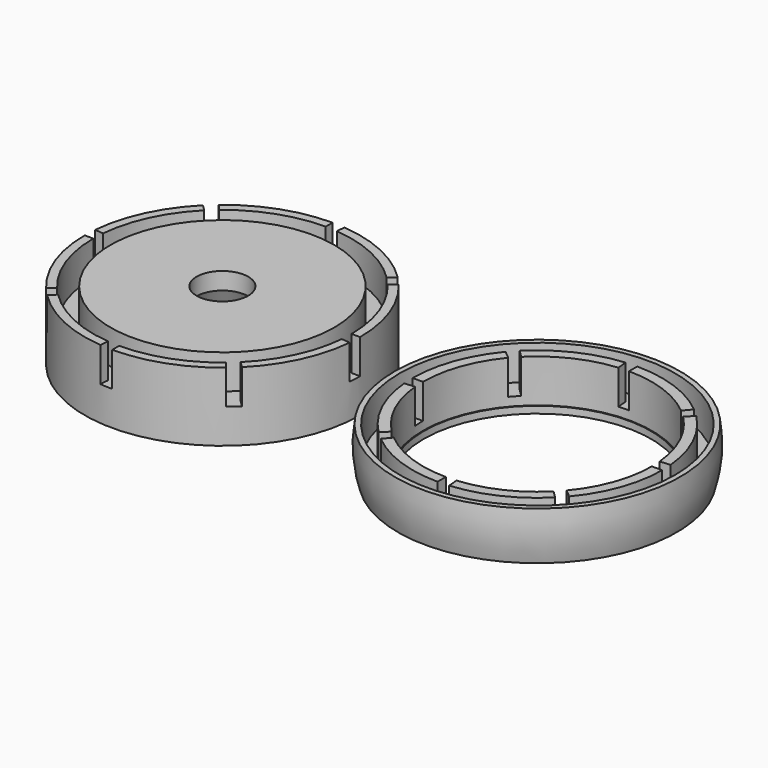
from build123d import *

# Parameters (mm, degrees)
F3_DEPTH        = 2.54
F3_COPIES_COUNT = 8
F7_DEPTH        = 2.54
F7_COPIES_COUNT = 8


# Not quite as in the source:
# - a pattern or mirror of a feature is missing from the dataset's text; its kind, count and spacing are read off the source's solid


with BuildPart() as f1:
    # F0 (on Front) → F1 (revolve)
    with BuildSketch(Plane.XZ):
        Polygon((-6.35, 0), (0, 0), (0, 5.08), (-0.635, 5.08), (-0.635, 2.54), (-1.905, 2.54), (-1.905, 5.08), (-8.255, 5.08), (-8.255, 3.81), align=None)
    revolve(axis=Axis((-10.16, 0, 2.5961052161), (0, 0, 1)))

    # F2 (on face) → F3 (cut, through all)
    with BuildSketch(Plane.XY.offset(5.08)):
        with BuildLine():
            ThreePointArc((-0.635, 0), (-0.6445944791, -0.4274140533), (-0.6733585875, -0.853967043))
            Line((-0.6733585875, -0.853967043), (-0.0409158267, -0.9108981792))
            ThreePointArc((-0.0409158267, -0.9108981792), (-0.010234111, -0.4559083235), (0, 0))
            Line((0, 0), (-0.635, 0))
        make_face()
    f3 = extrude(amount=-F3_DEPTH, mode=Mode.SUBTRACT)

    # F3_copies: F3 ×8 about axis
    f3_copies_axis = Axis((-10.16, 0, 0), (0, 0, 1))
    for i in range(1, F3_COPIES_COUNT):
        add(f3.rotate(f3_copies_axis, i * 360 / F3_COPIES_COUNT), mode=Mode.SUBTRACT)


with BuildPart() as f5:
    # F4 (on Front) → F5 (revolve)
    with BuildSketch(Plane.XZ):
        with BuildLine():
            Line((2.794, 0), (4.699, 0))
            Line((4.699, 0), (4.699, 0.508))
            Line((4.699, 0.508), (4.6355, 0.508))
            Line((4.6355, 0.508), (4.6355, 3.683))
            Line((4.6355, 3.683), (3.8735, 3.683))
            Line((3.8735, 3.683), (3.8735, 1.143))
            Line((3.8735, 1.143), (2.921, 1.143))
            Line((2.921, 1.143), (2.921, 3.683))
            Line((2.921, 3.683), (2.54, 3.683))
            ThreePointArc((2.54, 3.683), (2.4478454241, 1.8263858913), (2.794, 0))
        make_face()
    revolve(axis=Axis((13.081, 0, 1.3761192095), (0, 0, 1)))

    # F6 (on face) → F7 (cut, through all)
    with BuildSketch(Plane.XY.offset(3.683)):
        with BuildLine():
            ThreePointArc((12.3236263902, 8.4114716587), (12.7019311696, 8.4369886258), (13.081, 8.4455))
            Line((13.081, 8.4455), (13.081, 9.2075))
            ThreePointArc((13.081, 9.2075), (12.6677294706, 9.1982206823), (12.2552919292, 9.1704014324))
            Line((12.2552919292, 9.1704014324), (12.3236263902, 8.4114716587))
        make_face()
    f7 = extrude(amount=-F7_DEPTH, mode=Mode.SUBTRACT)

    # F7_copies: F7 ×8 about axis
    f7_copies_axis = Axis((13.081, 0, 0), (0, 0, 1))
    for i in range(1, F7_COPIES_COUNT):
        add(f7.rotate(f7_copies_axis, i * 360 / F7_COPIES_COUNT), mode=Mode.SUBTRACT)


solid = Compound([f1.part, f5.part])
